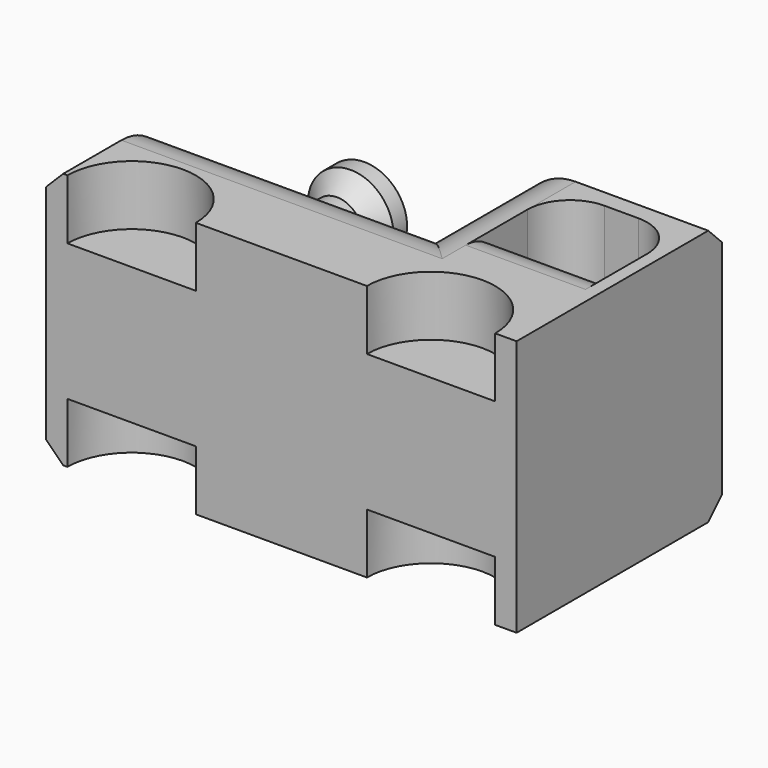
from build123d import *

# Parameters (mm, degrees)
F1_DEPTH  = 15
F3_DEPTH  = 7
F4_R      = 6.5
F5_SIZE   = 2
F6_W      = 14
F6_H      = 9
F7_DEPTH  = 30.001
F8_R      = 5
F9_R      = 3
F10_DEPTH = 1
F11_R     = 3
F12_DEPTH = 15
F13_R     = 5
F14_DEPTH = 4
F15_SIZE  = 1.99999


# Not quite as in the source:
# - a fillet or chamfer is up to 0.001 mm smaller than in the source, because OpenCascade refuses the exact size
# - a pattern or mirror of a feature is missing from the dataset's text; its kind, count and spacing are read off the source's solid


with BuildPart() as f1:
    # F0 (on Top) → F1 (new body, symmetric)
    with BuildSketch(Plane.XY):
        Polygon((27.5, 15), (5.5, 15), (5.5, 0), (-27.5, 0), (-27.5, -15), (27.5, -15), align=None)
    extrude(amount=F1_DEPTH, both=True)

    # F2 (on face) → F3 (cut)
    with BuildSketch(Plane.XY.offset(15)):
        with BuildLine():
            Line((-25, -15), (-10, -15))
            ThreePointArc((-10, -15), (-17.5, -7.5), (-25, -15))
        make_face()
        with BuildLine():
            ThreePointArc((25, -15), (17.5, -7.5), (10, -15))
            Line((10, -15), (25, -15))
        make_face()
    f3 = extrude(amount=-F3_DEPTH, mode=Mode.SUBTRACT)

    # F3_copies: F3 across plane
    add(f3.mirror(Plane(origin=(0, 0, 0), x_dir=(-1, 0, 0), z_dir=(0, 0, -1))), mode=Mode.SUBTRACT)

    # F4
    f4_edges = [f1.edges().sort_by_distance(p)[0] for p in [
        (-11, 0, 15),
        (-11, 0, -15),
        (5.5, 7.5, 15),
        (5.5, 7.5, -15),
    ]]
    fillet(f4_edges, radius=F4_R)

    # F5
    f5_edges = [f1.edges().sort_by_distance(p)[0] for p in [
        (5.5, 15, 0),
        (-27.5, 0, 0),
    ]]
    chamfer(f5_edges, length=F5_SIZE)

    # F6 (on face) → F7 (cut, through all)
    with BuildSketch(Plane.XY.offset(15)):
        with Locations((19.0077603161, 6.4331619842)):
            Rectangle(F6_W, F6_H)
    extrude(amount=-F7_DEPTH, mode=Mode.SUBTRACT)

    # F8
    f8_edges = [f1.edges().sort_by_distance(p)[0] for p in [
        (19.00776, 1.933162, 15),
        (26.00776, 10.933162, 0),
        (12.00776, 10.933162, 0),
    ]]
    fillet(f8_edges, radius=F8_R)

    # F9 (on face) → F10 (join)
    with BuildSketch(Plane(origin=(-27.5, 0, 0), x_dir=(0, -1, 0), z_dir=(-1, 0, 0))):
        with Locations((6.5, 8.5)):
            Circle(F9_R)
        with Locations((6.5, -8.5)):
            Circle(F9_R)
    extrude(amount=F10_DEPTH)

    # F11 (on face) → F12 (join)
    with BuildSketch(Plane(origin=(0, 0, 0), x_dir=(-1, 0, 0), z_dir=(0, 1, 0))):
        with Locations((17.5, 0)):
            Circle(F11_R)
    extrude(amount=F12_DEPTH)

    # F13 (on face) → F14 (join)
    with BuildSketch(Plane(origin=(0, 15, 0), x_dir=(-1, 0, 0), z_dir=(0, 1, 0))):
        with Locations((17.5, 0)):
            Circle(F13_R)
    extrude(amount=F14_DEPTH)

    # F15 (size 2 in the source; OpenCascade refuses exactly that, so slightly less here)
    f15_edges = [f1.edges().sort_by_distance(p)[0] for p in [
        (-12.5, 15, 0),
    ]]
    chamfer(f15_edges, length=F15_SIZE)


solid = f1.part
